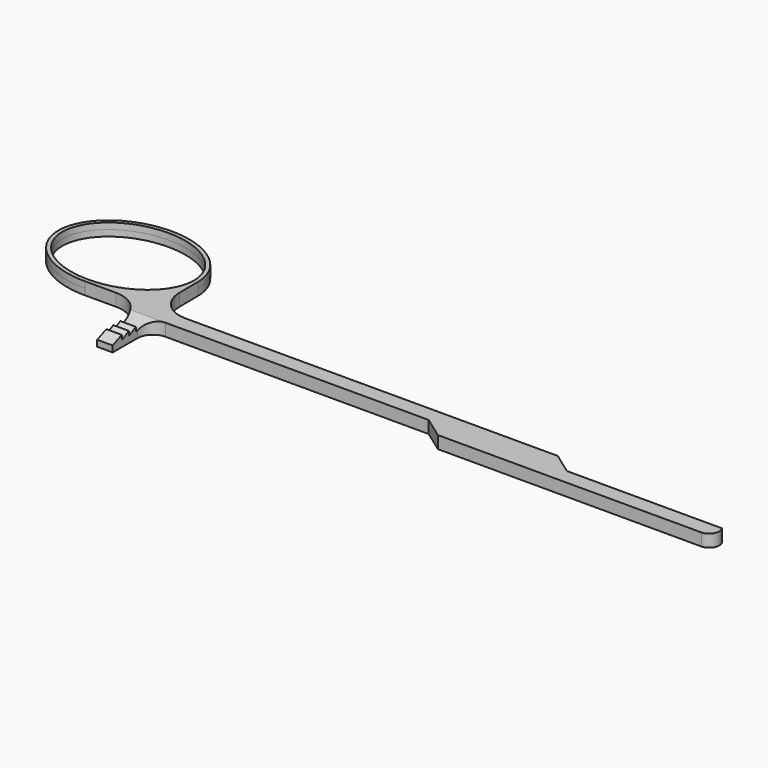
from build123d import *

# Parameters (mm, degrees)
F1_DEPTH      = 1.27
F1_DEPTH_BACK = 1.27
F3_DEPTH      = 6.0699698694
F4_DEPTH      = 26.9885001


# Not quite as in the source:
# - a feature names something its author has since deleted; it is built from what else it names


with BuildPart() as f1:
    # F0 (on Top) → F1 (new body, two sides)
    with BuildSketch(Plane.XY) as f1_sk:
        with BuildLine():
            Line((28.36282759, 0), (26.0949704471, -3.175))
            Line((26.0949704471, -3.175), (58.42, -3.175))
            ThreePointArc((58.42, -3.175), (60.2190476821, -2.0954196621), (60.11282759, 0))
            Line((60.11282759, 0), (28.36282759, 0))
        make_face()
        Polygon((-1.27, 0), (0, 0), (4.445, -3.175), (26.0949704471, -3.175), (28.36282759, 0), (23.91782759, 0), (23.91782759, 3.175), (0, 3.175), align=None)
        Polygon((28.36282759, 0), (23.91782759, 3.175), (23.91782759, 0), align=None)
        with BuildLine():
            add(Edge.make_bspline(
                [(-73.025, 3.175), (-58.7375, 3.175), (-58.7375, 14.2875)],
                knots=[1.5707963268, 1.5707963268, 1.5707963268, 3.1415926536, 3.1415926536, 3.1415926536], degree=2, weights=[1, 0.7071067812, 1]))
            add(Edge.make_bspline(
                [(-58.7375, 14.2875), (-58.7375, 25.4), (-73.025, 25.4)],
                knots=[3.1415926536, 3.1415926536, 3.1415926536, 4.7123889804, 4.7123889804, 4.7123889804], degree=2, weights=[1, 0.7071067812, 1]))
            Line((-73.025, 25.4), (-73.025, 24.60625))
            add(Edge.make_bspline(
                [(-73.025, 3.96875), (-59.53125, 3.96875), (-59.53125, 14.2875), (-59.53125, 24.60625), (-73.025, 24.60625)],
                knots=[1.5707963268, 1.5707963268, 1.5707963268, 3.1415926536, 3.1415926536, 4.7123889804, 4.7123889804, 4.7123889804], degree=2, weights=[1, 0.7071067812, 1, 0.7071067812, 1]))
            Line((-73.025, 3.96875), (-73.025, 3.175))
        make_face()
        with BuildLine():
            add(Edge.make_bspline(
                [(-73.025, 25.4), (-87.3125, 25.4), (-87.3125, 14.2875), (-87.3125, 3.175), (-73.025, 3.175)],
                knots=[4.7123889804, 4.7123889804, 4.7123889804, 6.2831853072, 6.2831853072, 7.853981634, 7.853981634, 7.853981634], degree=2, weights=[1, 0.7071067812, 1, 0.7071067812, 1]))
            Line((-73.025, 3.175), (-73.025, 3.96875))
            add(Edge.make_bspline(
                [(-73.025, 24.60625), (-86.51875, 24.60625), (-86.51875, 14.2875), (-86.51875, 3.96875), (-73.025, 3.96875)],
                knots=[4.7123889804, 4.7123889804, 4.7123889804, 6.2831853072, 6.2831853072, 7.853981634, 7.853981634, 7.853981634], degree=2, weights=[1, 0.7071067812, 1, 0.7071067812, 1]))
            Line((-73.025, 24.60625), (-73.025, 25.4))
        make_face()
        with BuildLine():
            Line((-53.975, 0), (-1.27, 0))
            Line((-1.27, 0), (0, 3.175))
            Line((0, 3.175), (-52.3420743746, 3.175))
            ThreePointArc((-52.3420743746, 3.175), (-56.8108733454, 5.0136436897), (-58.6917891577, 9.4648155091))
            Line((-58.6917891577, 9.4648155091), (-58.7375, 14.2875))
            add(Edge.make_bspline(
                [(-73.025, 3.175), (-58.7375, 3.175), (-58.7375, 14.2875)],
                knots=[1.5707963268, 1.5707963268, 1.5707963268, 3.1415926536, 3.1415926536, 3.1415926536], degree=2, weights=[1, 0.7071067812, 1]))
            Line((-73.025, 3.175), (-66.675, 3.175))
            ThreePointArc((-66.675, 3.175), (-62.1848719395, 1.3151280605), (-60.325, -3.175))
            Line((-60.325, -3.175), (-60.325, -9.525))
            Line((-60.325, -9.525), (-57.15, -9.525))
            Line((-57.15, -9.525), (-57.15, -3.175))
            ThreePointArc((-57.15, -3.175), (-56.2200640303, -0.9299359697), (-53.975, 0))
        make_face()
    extrude(amount=F1_DEPTH)
    extrude(f1_sk.sketch, amount=-F1_DEPTH_BACK)

    # F2 (on face) → F3 (cut, through all)
    with BuildSketch(Plane(origin=(-60.325, 0, 0), x_dir=(0, -1, 0), z_dir=(-1, 0, 0))):
        Polygon((3.175, 1.27), (3.175, 0.1474900148), (3.590535535, 0), (3.590535535, 0.9525), (5.3854638761, 0), (5.3854638761, 0.9525), (7.1803922173, 0), (7.1803922173, 0.9525), (9.525, 0), (9.525, 1.27), align=None)
        Polygon((9.525, 1.27), (0, 1.2744232312), (3.175, 0.1474900148), (3.175, 1.27), align=None)
    extrude(amount=-F3_DEPTH, mode=Mode.SUBTRACT)

    # F4 (cut, through all): a face of the model
    f4_faces = [f1.faces().sort_by_distance(p)[0] for p in [
        (-60.325, -2.1208206422, 0.8958300049),
    ]]
    extrude(f4_faces, amount=-F4_DEPTH, mode=Mode.SUBTRACT)


solid = f1.part
